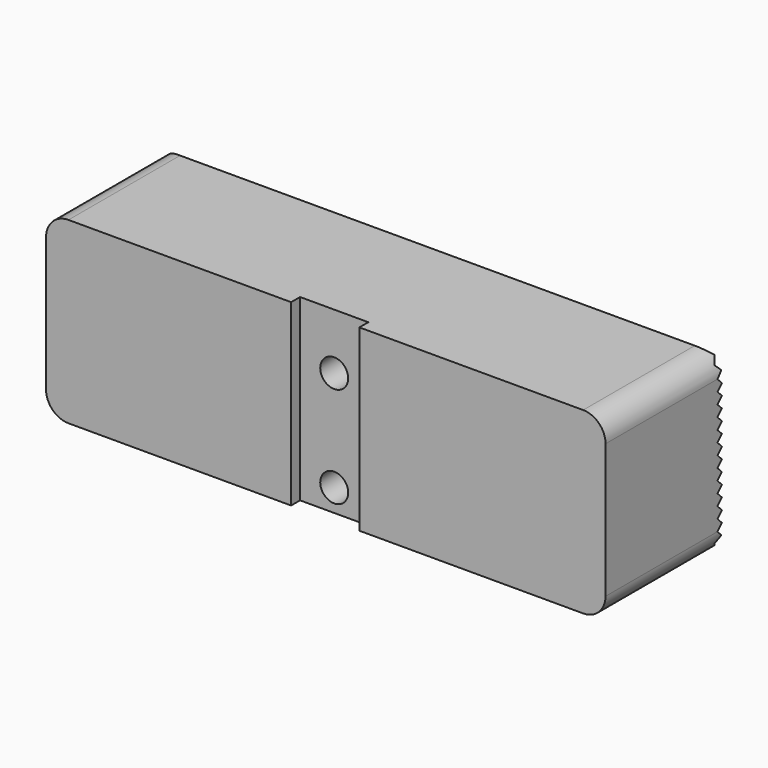
from build123d import *

# Parameters (mm, degrees)
F0_W         = 50
F0_H         = 16
F1_DEPTH     = 13
F2_W         = 6.1
F2_H         = 2
F2_H_2       = 16
F3_DEPTH     = 1
F5_D         = 2.5
F5_DEPTH     = 9.5
F5_TIP       = 0.7510757738
F6_SIZE      = 0.5
F8_DEPTH     = 50.001
F9_DEPTH     = 50.001
F10_T1_DEPTH = 22.4650386507
F10_T3_DEPTH = 22.5


# Not quite as in the source:
# - a fillet or chamfer that OpenCascade refuses, or shapes differently, is made with other operations: its cross-section is extruded or revolved along the edge and cut away or added


with BuildPart() as f1:
    # F0 (on Front) → F1 (new body)
    with BuildSketch(Plane.XZ):
        with Locations((25, 8)):
            Rectangle(F0_W, F0_H)
    extrude(amount=F1_DEPTH)

    # F2 (on face) → F3 (cut)
    with BuildSketch(Plane.XZ.offset(13)):
        with Locations((24.95, -1)):
            Rectangle(F2_W, F2_H)
        with Locations((24.95, 8)):
            Rectangle(F2_W, F2_H_2)
    extrude(amount=-F3_DEPTH, mode=Mode.SUBTRACT)

    # F5
    with Locations(Plane.XZ.offset(12)):
        with Locations((24.95, 11), (24.95, 2)):
            Hole(F5_D / 2, depth=F5_DEPTH)
            with Locations((0, 0, -(F5_DEPTH + F5_TIP / 2))):  # 118° drill point
                Cone(0, F5_D / 2, F5_TIP, mode=Mode.SUBTRACT)

    # F6
    f6_edges = [f1.edges().sort_by_distance(p)[0] for p in [
        (0, 0, 8),
        (25, 0, 16),
        (25, 0, 0),
    ]]
    chamfer(f6_edges, length=F6_SIZE)

    # F7 (on face) → F8 (cut, through all)
    with BuildSketch(Plane(origin=(0, 0, 0), x_dir=(0, -1, 0), z_dir=(-1, 0, 0))):
        Polygon((0, 3.5), (0, 2.5), (0.5, 3), align=None)
        Polygon((0, 4.5), (0, 3.5), (0.5, 4), align=None)
        Polygon((0, 5.5), (0, 4.5), (0.5, 5), align=None)
        Polygon((0, 6.5), (0, 5.5), (0.5, 6), align=None)
        Polygon((0, 7.5), (0, 6.5), (0.5, 7), align=None)
        Polygon((0, 8.5), (0, 7.5), (0.5, 8), align=None)
        Polygon((0, 9.5), (0, 8.5), (0.5, 9), align=None)
        Polygon((0, 10.5), (0, 9.5), (0.5, 10), align=None)
        Polygon((0, 11.5), (0, 10.5), (0.5, 11), align=None)
        Polygon((0.5, 12), (0, 12.5), (0, 11.5), align=None)
        Polygon((0.5, 13), (0, 13.5), (0, 12.5), align=None)
        Polygon((0.5, 14), (0, 14.5), (0, 13.5), align=None)
        Polygon((0.5, 15), (0, 15.5), (0, 14.5), align=None)
        Polygon((0.5, 16), (0.5349613493, 16), (0, 16.5), (0, 15.5), (0.5, 15.9673234811), align=None)
        Polygon((0.5, 15.9673234811), (0.5349613493, 16), (0.5, 16), align=None)
        Polygon((0, 1.5), (0, 0.5), (0.5, 1), align=None)
    extrude(amount=-F8_DEPTH, mode=Mode.SUBTRACT)

    # F7 (on face) → F9 (cut, through all)
    with BuildSketch(Plane(origin=(0, 0, 0), x_dir=(0, -1, 0), z_dir=(-1, 0, 0))):
        Polygon((0, 2.5), (0, 1.5), (0.5, 2), align=None)
    extrude(amount=-F9_DEPTH, mode=Mode.SUBTRACT)

    # F10: fillet of radius 2 on 4 edges, made by hand

    # F10_s2 → F10_t1 (cut)
    with BuildSketch(Plane.XZ.offset(-4.4650386507)):
        with BuildLine():
            ThreePointArc((48, 16), (49.4142135624, 15.4142135624), (50, 14))
            Line((50, 14), (50, 16))
            Line((50, 16), (48, 16))
        make_face()
        with BuildLine():
            ThreePointArc((0, 14), (0.5857864376, 15.4142135624), (2, 16))
            Line((2, 16), (0, 16))
            Line((0, 16), (0, 14))
        make_face()
    extrude(amount=F10_T1_DEPTH, mode=Mode.SUBTRACT)

    # F10_s4 → F10_t3 (cut)
    with BuildSketch(Plane.XZ.offset(-4.5)):
        with BuildLine():
            ThreePointArc((48, 0), (49.4142135624, 0.5857864376), (50, 2))
            Line((50, 2), (50, 0))
            Line((50, 0), (48, 0))
        make_face()
        with BuildLine():
            ThreePointArc((0, 2), (0.5857864376, 0.5857864376), (2, 0))
            Line((2, 0), (0, 0))
            Line((0, 0), (0, 2))
        make_face()
    extrude(amount=F10_T3_DEPTH, mode=Mode.SUBTRACT)


solid = f1.part
